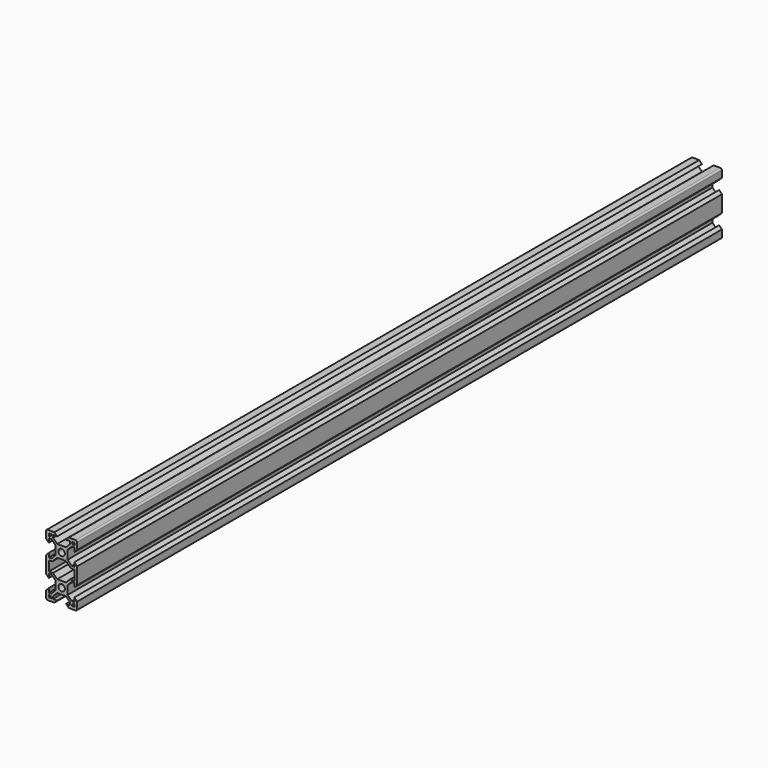
from build123d import *

# Parameters (mm, degrees)
F0_W             = 20
F0_H             = 20
F1_DEPTH         = 520
F2_R             = 2.1
F3_DEPTH         = 520.001
F4_R             = 1
F6_DEPTH         = 520.001
F6_COPIES3_COUNT = 2
F6_COPIES3_ANGLE = 90
F6_COPIES4_COUNT = 2
F6_COPIES4_ANGLE = 270
F6_COPIES6_COUNT = 2
F9_W             = 16.4
F9_H             = 6.8613203436
F10_DEPTH        = 520.001
F12_DEPTH        = 520


# Not quite as in the source:
# - a pattern or mirror of a feature is missing from the dataset's text; its kind, count and spacing are read off the source's solid


with BuildPart() as f1:
    # F0 (on Front) → F1 (new body)
    with BuildSketch(Plane.XZ):
        Rectangle(F0_W, F0_H)
    extrude(amount=F1_DEPTH)

    # F2 (on face) → F3 (cut, through all)
    with BuildSketch(Plane.XZ.offset(520)):
        Circle(F2_R)
    extrude(amount=-F3_DEPTH, mode=Mode.SUBTRACT)

    # F4
    f4_edges = [f1.edges().sort_by_distance(p)[0] for p in [
        (-10, -260, 10),
        (10, -260, 10),
    ]]
    fillet(f4_edges, radius=F4_R)

    # F5 (on face) → F6 (cut, through all)
    with BuildSketch(Plane.XZ.offset(520)):
        Polygon((0, 3.9006601718), (0, 10), (-2.84, 10), (-4.64, 10), (-2.84, 8.2), (-5.4993398282, 8.2), (-5.4993398282, 6.56), (-2.84, 3.9006601718), align=None)
        Polygon((-6.5693398282, 8.2), (-8.2, 8.2), (-7.0953059148, 7.0953059148), (-6.5693398282, 7.6212720014), align=None)
    f6 = extrude(amount=-F6_DEPTH, mode=Mode.SUBTRACT)

    # F6_copies: F6 across plane
    add(f6.mirror(Plane(origin=(0, 0, 0), x_dir=(-0.7071067812, 0, -0.7071067812), z_dir=(0.7071067812, 0, -0.7071067812))), mode=Mode.SUBTRACT)

    # F6_copies1: F6 across plane
    add(f6.mirror(Plane(origin=(0, 0, 0), x_dir=(0.7071067812, 0, -0.7071067812), z_dir=(-0.7071067812, 0, -0.7071067812))), mode=Mode.SUBTRACT)

    # F6_copies2: F6 across plane
    add(f6.mirror(Plane(origin=(0, 0, 0), x_dir=(0, 0, 1), z_dir=(1, 0, 0))), mode=Mode.SUBTRACT)

    # F6_copies3: F6 ×2 about axis
    f6_copies3_axis = Axis((0, 0, 0), (0, 1, 0))
    for i in range(1, F6_COPIES3_COUNT):
        add(f6.rotate(f6_copies3_axis, i * F6_COPIES3_ANGLE / (F6_COPIES3_COUNT - 1)), mode=Mode.SUBTRACT)

    # F6_copies4: F6 ×2 about axis
    f6_copies4_axis = Axis((0, 0, 0), (0, 1, 0))
    for i in range(1, F6_COPIES4_COUNT):
        add(f6.rotate(f6_copies4_axis, i * F6_COPIES4_ANGLE / (F6_COPIES4_COUNT - 1)), mode=Mode.SUBTRACT)

    # F6_copies5: F6 across plane
    add(f6.mirror(Plane(origin=(0, 0, 0), x_dir=(-1, 0, 0), z_dir=(0, 0, -1))), mode=Mode.SUBTRACT)

    # F6_copies6: F6 ×2 about axis
    f6_copies6_axis = Axis((0, 0, 0), (0, 1, 0))
    for i in range(1, F6_COPIES6_COUNT):
        add(f6.rotate(f6_copies6_axis, i * 360 / F6_COPIES6_COUNT), mode=Mode.SUBTRACT)

    # F8: F1 across face


with BuildPart() as f1_1:
    add(f1.part)
    add(f1.part.mirror(Plane(origin=(-7.32, -260, -10), x_dir=(1, 0, 0), z_dir=(0, 0, -1))))

    # F9 (on face) → F10 (cut, through all)
    with BuildSketch(Plane.XZ.offset(520)):
        with Locations((0, -10)):
            Rectangle(F9_W, F9_H)
    extrude(amount=-F10_DEPTH, mode=Mode.SUBTRACT)

    # F11 (on face) → F12 (join, through all)
    with BuildSketch(Plane.XZ.offset(520)):
        with BuildLine():
            ThreePointArc((-9, -10), (-9.7071067812, -9.7071067812), (-10, -9))
            Line((-10, -9), (-10, -11))
            ThreePointArc((-10, -11), (-9.7071067812, -10.2928932188), (-9, -10))
        make_face()
        with BuildLine():
            ThreePointArc((10, -9), (9.7071067812, -9.7071067812), (9, -10))
            ThreePointArc((9, -10), (9.7071067812, -10.2928932188), (10, -11))
            Line((10, -11), (10, -9))
        make_face()
        Polygon((5.9386796564, -6.9993398282), (8.2, -6.9993398282), (8.2, -6.5693398282), (5.5086796564, -6.5693398282), align=None)
        Polygon((-8.2, -6.5693398282), (-8.2, -6.9993398282), (-5.9386796564, -6.9993398282), (-5.5086796564, -6.5693398282), align=None)
    extrude(amount=-F12_DEPTH)


solid = f1_1.part
